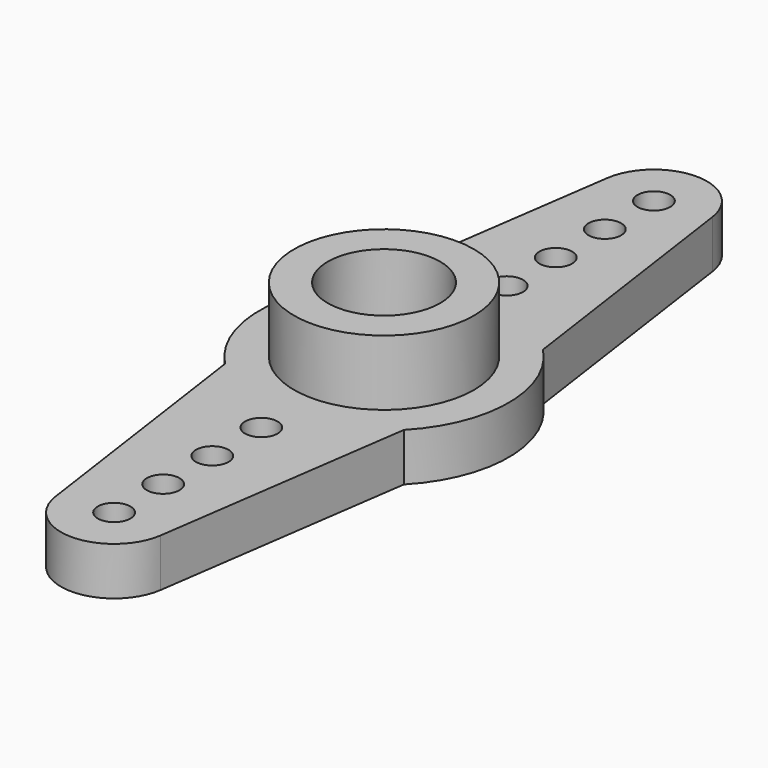
from build123d import *

# Parameters (mm, degrees)
F0_R     = 6.1
F0_R_2   = 4.4
F0_R_3   = 2.75
F0_R_4   = 1.45
F1_DEPTH = 2.35
F2_DEPTH = 5.55
F3_R     = 0.8
F4_DEPTH = 2.35
F6_R     = 4.5
F6_R_2   = 3.4
F6_R_3   = 2.9
F7_DEPTH = 0.7


# Not quite as in the source:
# - a pattern or mirror of a feature is missing from the dataset's text; its kind, count and spacing are read off the source's solid


with BuildPart() as f1:
    # F0 (on Top) → F1 (new body)
    with BuildSketch(Plane.XY):
        Circle(F0_R)
        Circle(F0_R_2, mode=Mode.SUBTRACT)
        Circle(F0_R_2)
        Circle(F0_R_3, mode=Mode.SUBTRACT)
        Circle(F0_R_3)
        Circle(F0_R_4, mode=Mode.SUBTRACT)
    extrude(amount=F1_DEPTH)

    # F0 (on Top) → F2 (join)
    with BuildSketch(Plane.XY):
        Circle(F0_R_2)
        Circle(F0_R_3, mode=Mode.SUBTRACT)
    extrude(amount=F2_DEPTH)

    # F3 (on Top) → F4 (join, through all)
    with BuildSketch(Plane.XY):
        with BuildLine():
            Line((-2.5739052597, 16.8674394022), (-4.375, 4.2508087466))
            ThreePointArc((-4.375, 4.2508087466), (0, 6.1), (4.375, 4.2508087466))
            Line((4.375, 4.2508087466), (2.5739052597, 16.8674394022))
            ThreePointArc((2.5739052597, 16.8674394022), (0, 19.1), (-2.5739052597, 16.8674394022))
        make_face()
        with Locations((0, 7.5)):
            Circle(F3_R, mode=Mode.SUBTRACT)
        with Locations((0, 10.5)):
            Circle(F3_R, mode=Mode.SUBTRACT)
        with Locations((0, 13.5)):
            Circle(F3_R, mode=Mode.SUBTRACT)
        with Locations((0, 16.5)):
            Circle(F3_R, mode=Mode.SUBTRACT)
    f4 = extrude(amount=F4_DEPTH)

    # F4_copies: F4 across plane
    add(f4.mirror(Plane(origin=(0, 0, 0), x_dir=(0, 0, -1), z_dir=(0, -1, 0))))

    # F6 (on face) → F7 (cut)
    with BuildSketch(Plane(origin=(0, 0, 0), x_dir=(1, 0, 0), z_dir=(0, 0, -1))):
        Circle(F6_R)
        Circle(F6_R_2, mode=Mode.SUBTRACT)
        Circle(F6_R_3)
    extrude(amount=-F7_DEPTH, mode=Mode.SUBTRACT)


solid = f1.part
